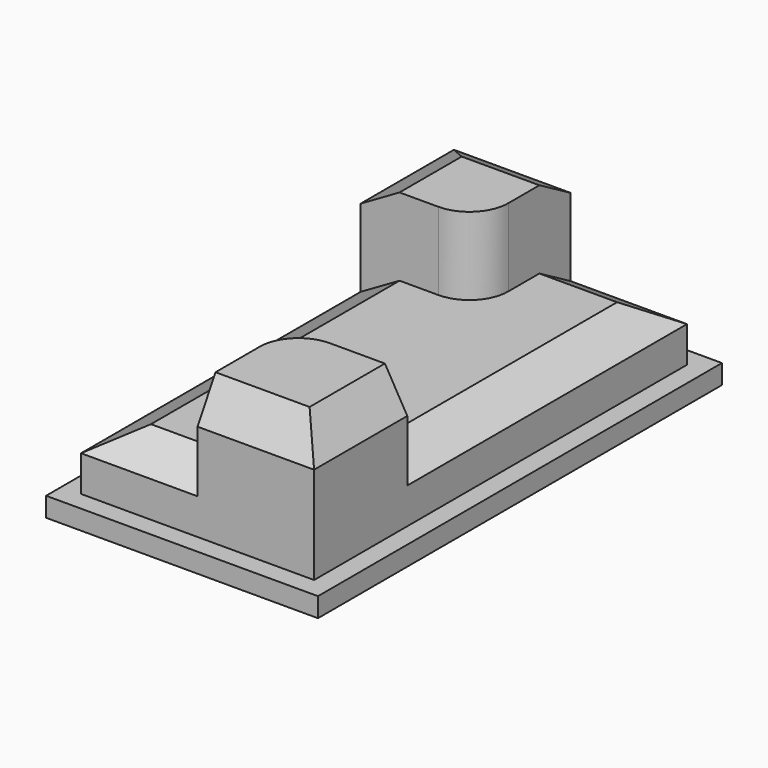
from build123d import *

# Parameters (mm, degrees)
F0_W        = 88.9
F0_H        = 165.1
F1_DEPTH    = 6.35
F2_DEPTH    = 25.4
F3_DEPTH    = 50.8
F4_SIZE2    = 7.3323484187
F4_SIZE     = 12.7
F5_C1_SIZE2 = 12.7
F5_C1_SIZE  = 7.3323484187
F5_C2_SIZE2 = 7.3323484187
F5_C2_SIZE  = 12.7
F5_C3_SIZE2 = 12.7
F5_C3_SIZE  = 7.3323484187
F5_C4_SIZE2 = 7.3323484187
F5_C4_SIZE  = 12.7


with BuildPart() as f1:
    # F0 (on Top) → F1 (new body)
    with BuildSketch(Plane.XY):
        Rectangle(F0_W, F0_H)
        Polygon((0, 76.2), (38.1, 76.2), (38.1, -38.1), (38.1, -76.2), (0, -76.2), (-38.1, -76.2), (-38.1, 38.1), (-38.1, 76.2), align=None, mode=Mode.SUBTRACT)
    extrude(amount=F1_DEPTH)

    # F0 (on Top) → F2 (join)
    with BuildSketch(Plane.XY):
        with BuildLine():
            Line((38.1, -38.1), (38.1, 76.2))
            Line((38.1, 76.2), (0, 76.2))
            Line((0, 76.2), (0, 50.8))
            ThreePointArc((0, 50.8), (-3.7197438789, 41.8197438789), (-12.7, 38.1))
            Line((-12.7, 38.1), (-38.1, 38.1))
            Line((-38.1, 38.1), (-38.1, -76.2))
            Line((-38.1, -76.2), (0, -76.2))
            Line((0, -76.2), (0, -50.8))
            ThreePointArc((0, -50.8), (3.7197438789, -41.8197438789), (12.7, -38.1))
            Line((12.7, -38.1), (38.1, -38.1))
        make_face()
    extrude(amount=F2_DEPTH)

    # F0 (on Top) → F3 (join)
    with BuildSketch(Plane.XY):
        with BuildLine():
            Line((0, 50.8), (0, 76.2))
            Line((0, 76.2), (-38.1, 76.2))
            Line((-38.1, 76.2), (-38.1, 38.1))
            Line((-38.1, 38.1), (-12.7, 38.1))
            ThreePointArc((-12.7, 38.1), (-3.7197438789, 41.8197438789), (0, 50.8))
        make_face()
        with BuildLine():
            Line((38.1, -76.2), (38.1, -38.1))
            Line((38.1, -38.1), (12.7, -38.1))
            ThreePointArc((12.7, -38.1), (3.7197438789, -41.8197438789), (0, -50.8))
            Line((0, -50.8), (0, -76.2))
            Line((0, -76.2), (38.1, -76.2))
        make_face()
    extrude(amount=F3_DEPTH)

    # F4
    f4_edges = [f1.edges().sort_by_distance(p)[0] for p in [
        (-38.1, -19.05, 25.4),
        (19.05, 76.2, 25.4),
        (38.1, 19.05, 25.4),
        (-19.05, -76.2, 25.4),
    ]]
    f4_side = f1.faces().sort_by_distance((0, 0, 25.4))[0]
    chamfer(f4_edges, length=F4_SIZE, length2=F4_SIZE2, reference=f4_side)

    # F5: chamfer of 12.7 x 7.3323484187 on 4 edges, made by hand

    # F5_c1
    f5_c1_edges = [f1.edges().sort_by_distance(p)[0] for p in [
        (-38.1, 57.15, 50.8),
    ]]
    f5_c1_side = f1.faces().sort_by_distance((-38.1, 57.15, 50.6533530316))[0]
    chamfer(f5_c1_edges, length=F5_C1_SIZE, length2=F5_C1_SIZE2, reference=f5_c1_side)

    # F5_c2
    f5_c2_edges = [f1.edges().sort_by_distance(p)[0] for p in [
        (19.05, -76.2, 50.8),
    ]]
    f5_c2_side = f1.faces().sort_by_distance((19.05, -76.2, 50.6533530316))[0]
    chamfer(f5_c2_edges, length=F5_C2_SIZE, length2=F5_C2_SIZE2, reference=f5_c2_side)

    # F5_c3
    f5_c3_edges = [f1.edges().sort_by_distance(p)[0] for p in [
        (-12.7, 76.2, 50.8),
    ]]
    f5_c3_side = f1.faces().sort_by_distance((-12.7, 76.2, 50.6533530316))[0]
    chamfer(f5_c3_edges, length=F5_C3_SIZE, length2=F5_C3_SIZE2, reference=f5_c3_side)

    # F5_c4
    f5_c4_edges = [f1.edges().sort_by_distance(p)[0] for p in [
        (38.1, -53.4838257906, 50.8),
    ]]
    f5_c4_side = f1.faces().sort_by_distance((38.1, -53.4838257906, 50.6533530316))[0]
    chamfer(f5_c4_edges, length=F5_C4_SIZE, length2=F5_C4_SIZE2, reference=f5_c4_side)


solid = f1.part
